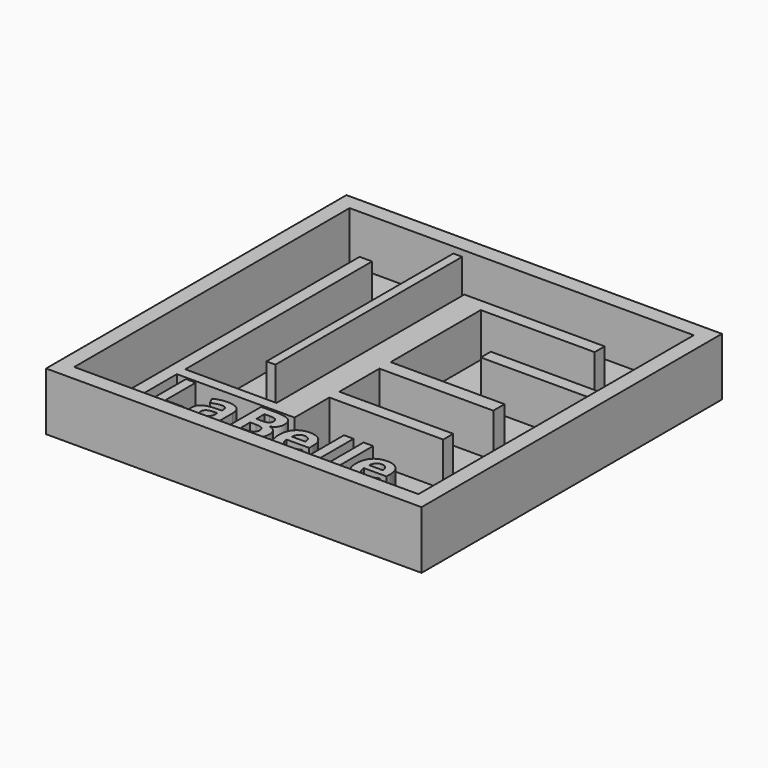
from build123d import *

# Parameters (mm, degrees)
F0_W         = 38.1
F0_H         = 38.1
F1_DEPTH     = 0.79375
F2_W         = 38.1
F2_H         = 38.1
F2_W_2       = 34.925
F2_H_2       = 34.925
F3_DEPTH     = 5.08
F4_W         = 0.904598192
F4_H         = 23.7001644473
F4_W_2       = 11.5564738645
F4_H_2       = 1.27
F4_TEXT_SIZE = 6.5263888889
F5_DEPTH     = 4.445
F6_R         = 1.27
F7_DEPTH     = 0.396875


# Not quite as in the source:
# - Text() gives the source's letters only with a copy of the font that has no kerning and outlines rounded to 1/6400 em; it was checked with that copy


with BuildPart() as f1:
    # F0 (on Top) → F1 (new body)
    with BuildSketch(Plane.XY):
        with Locations((1.857098192, -2.3782805847)):
            Rectangle(F0_W, F0_H)
    extrude(amount=F1_DEPTH)

    # F2 (on face) → F3 (join)
    with BuildSketch(Plane.XY.offset(0.79375)):
        with Locations((1.857098192, -2.3782805847)):
            Rectangle(F2_W, F2_H)
        with Locations((1.857098192, -2.3782805847)):
            Rectangle(F2_W_2, F2_H_2, mode=Mode.SUBTRACT)
    extrude(amount=F3_DEPTH)

    # F4 (on face) → F5 (join)
    with BuildSketch(Plane.XY.offset(0.79375)):
        Polygon((-10.525401808, 10.0042194153), (-10.525401808, -19.8407805847), (-9.255401808, -19.8407805847), (-9.255401808, -14.7607805847), (0, -14.7607805847), (2.6831243275, -14.7607805847), (2.6831243275, -10.3435385972), (14.239598192, -10.3435385972), (14.239598192, -9.0735385972), (2.6831243275, -9.0735385972), (2.6831243275, -3.9935385972), (14.239598192, -3.9935385972), (14.239598192, -2.5647832081), (2.6831243275, -2.5647832081), (2.6831243275, 8.8652167919), (14.239598192, 8.8652167919), (14.239598192, 10.1352167919), (2.6831243275, 10.1352167919), (0, 10.1352167919), (0, 10.0718266909), (0, -13.6959450319), (-9.255401808, -13.6959450319), (-9.255401808, 10.0042194153), align=None)
        with Locations((-4.627700904, 3.2341371917)):
            Rectangle(F4_W, F4_H)
        with Locations((13.5413612597, 3.1502167919)):
            Rectangle(F4_W_2, F4_H_2)
        with Locations((-8.7468111888, -19.6332687801)):
            Text('LaBelle', F4_TEXT_SIZE, font='Open Sans', font_style=FontStyle.BOLD, text_align=(TextAlign.LEFT, TextAlign.BOTTOM))
    extrude(amount=F5_DEPTH)

    # F6 (on face) → F7 (cut)
    with BuildSketch(Plane.XY.offset(0.79375)):
        with BuildLine():
            add(Edge.make_bspline(
                [(-3.9627806081, -16.1194378063), (-4.2180342393, -16.1956023193), (-4.4536709978, -16.3190869224)],
                knots=[2.6439921805, 2.6439921805, 2.6439921805, 3.0440967283, 3.0440967283, 3.0440967283], degree=2))
            ThreePointArc((-3.9627806081, -16.1194378063), (-6.3295493685, -16.357585225), (-4.388407062, -17.7324579843))
            ThreePointArc((-4.388407062, -17.7324579843), (-4.0239543928, -17.3536377156), (-3.8441262273, -16.8596818724))
            add(Edge.make_bspline(
                [(-4.1324502947, -16.9758048044), (-3.9832819868, -16.9091270979), (-3.8441262273, -16.8596818724)],
                knots=[0, 0, 0, 0.2584444185, 0.2584444185, 0.2584444185], degree=2))
            Line((-4.1324502947, -16.9758048044), (-4.4536709978, -16.3190869224))
        make_face()
        with Locations((5.8455416001, -6.5335385972)):
            Circle(F6_R)
    extrude(amount=-F7_DEPTH, mode=Mode.SUBTRACT)


solid = f1.part
